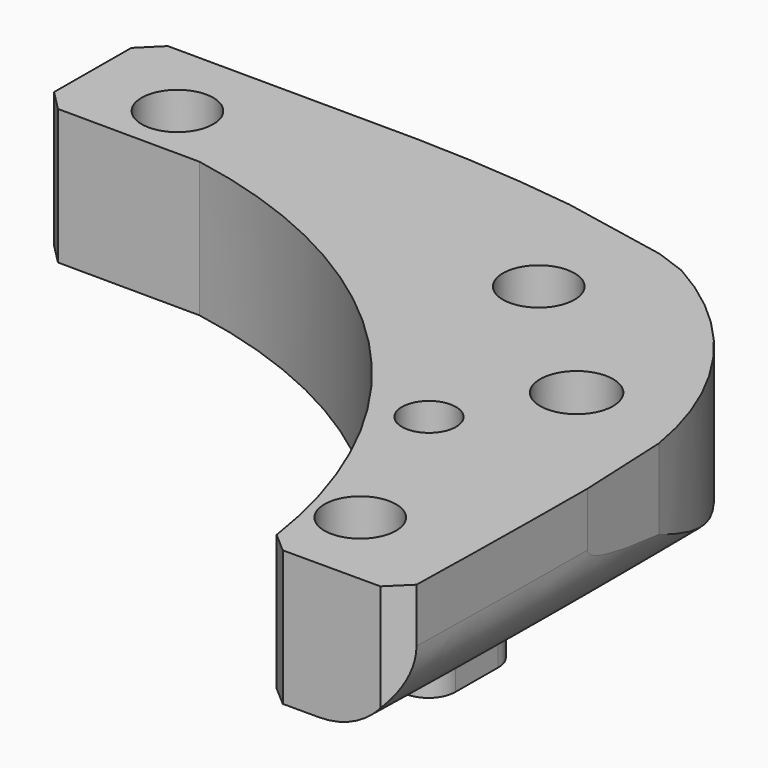
from build123d import *

# Parameters (mm, degrees)
F1_DEPTH    = 10
F2_R        = 2.65
F2_R_2      = 2.7
F3_DEPTH    = 10.001
F4_T2_ANGLE = 6.3743045961
F6_DEPTH    = 6
F7_R        = 2
F8_T1_DEPTH = 17.7150489639
F8_T3_DEPTH = 16.827176909
F8_T5_DEPTH = 14.1871505468
F9_T1_DEPTH = 16.8101610382
F10_R       = 2
F11_DEPTH   = 16


# Not quite as in the source:
# - a fillet or chamfer that OpenCascade refuses, or shapes differently, is made with other operations: its cross-section is extruded or revolved along the edge and cut away or added
# - a feature names something its author has since deleted; it is built from what else it names


with BuildPart() as f1:
    # F0 (on Top) → F1 (new body)
    with BuildSketch(Plane.XY):
        with BuildLine():
            Line((-34.7499609253, -11.2477834763), (-54.7499609253, -11.1477834763))
            Line((-54.7499609253, -11.1477834763), (-54.8004609253, -21.2477834763))
            Line((-54.8004609253, -21.2477834763), (-42.8006109225, -21.3077827264))
            ThreePointArc((-42.8006109225, -21.3077827264), (-20.5885311059, -33.3218659489), (-10, -56.2477834763))
            Line((-10, -56.2477834763), (0, -56.2477834763))
            ThreePointArc((0, -56.2477834763), (0.1673692192, -47.7484327866), (0.2444140549, -39.2477834763))
            Line((0.2444140549, -39.2477834763), (-0.07466726, -32.2477834763))
            ThreePointArc((-0.07466726, -32.2477834763), (-4.6744272783, -21.4152799032), (-13.7499609253, -13.9229094565))
            Line((-13.7499609253, -13.9229094565), (-22.7499609253, -12.1477834763))
            ThreePointArc((-22.7499609253, -12.1477834763), (-28.7364107349, -11.5171142711), (-34.7499609253, -11.2477834763))
        make_face()
    extrude(amount=F1_DEPTH)

    # F2 (on face) → F3 (cut, through all)
    with BuildSketch(Plane.XY.offset(10)):
        with Locations((-47.7499609253, -17.1477834763)):
            Circle(F2_R)
        with Locations((-17.7499609253, -21.2477834763)):
            Circle(F2_R)
        with Locations((-7.7499609253, -50.2477834763)):
            Circle(F2_R)
        with Locations((-7.7499609253, -30.2477834763)):
            Circle(F2_R_2)
    extrude(amount=-F3_DEPTH, mode=Mode.SUBTRACT)

    # F4: fillet of radius 6 on 1 edges, made by hand

    # F4_s1 → F4_t2 (revolve, cut)
    with BuildSketch(Plane(origin=(-6.441827323, -91.8723118046, 0), x_dir=(0, 0, 1), z_dir=(-0.0699454492, -0.9975508178, 0))):
        with BuildLine():
            ThreePointArc((0, 1.2558600799), (1.7573593129, -2.9867806073), (6, -4.7441399201))
            Line((6, -4.7441399201), (6, -4.8641399201))
            Line((6, -4.8641399201), (-0.12, -4.8641399201))
            Line((-0.12, -4.8641399201), (-0.12, 1.2558600799))
            Line((-0.12, 1.2558600799), (0, 1.2558600799))
        make_face()
    revolve(axis=Axis((-799.7499609255, -36.2477834763, 0), (0, 0, 1)), revolution_arc=F4_T2_ANGLE, mode=Mode.SUBTRACT)

    # F5 (on face) → F6 (join)
    with BuildSketch(Plane.XY):
        Polygon((-20, -32.2477834763), (-14.04, -41.3386925673), (-9.04, -42.2477834763), (-9, -34.2477834763), align=None)
    extrude(amount=-F6_DEPTH)

    # F7
    f7_edges = [f1.edges().sort_by_distance(p)[0] for p in [
        (-9, -34.247783, -3),
        (-20, -32.247783, -3),
        (-14.04, -41.338693, -3),
        (-9.04, -42.247783, -3),
    ]]
    fillet(f7_edges, radius=F7_R)

    # F8: chamfer of 1.5 on 4 edges, made by hand

    # F8_s2 → F8_t1 (cut)
    with BuildSketch(Plane.XY.offset(-3.8575244819)):
        Polygon((-53.2499796749, -11.1552833826), (-54.7574608315, -12.6477647267), (-54.7499609253, -11.1477834763), align=None)
        Polygon((-54.792961019, -19.747802226), (-53.3004796749, -21.2552833826), (-54.8004609253, -21.2477834763), align=None)
    extrude(amount=F8_T1_DEPTH, mode=Mode.SUBTRACT)

    # F8_s4 → F8_t3 (cut)
    with BuildSketch(Plane.XY.offset(-3.4135884545)):
        with BuildLine():
            Line((-10.1649915082, -54.9628953089), (-8.6804960049, -56.2477834763))
            Line((-8.6804960049, -56.2477834763), (-10, -56.2477834763))
            ThreePointArc((-10, -56.2477834763), (-10.0801500361, -55.5824778984), (-10.1649915082, -54.9628953089))
        make_face()
    extrude(amount=F8_T3_DEPTH, mode=Mode.SUBTRACT)

    # F8_s6 → F8_t5 (cut)
    with BuildSketch(Plane.XY.offset(-0.4141318258)):
        with BuildLine():
            Line((-1.4642977695, -56.2477834763), (0.0352995939, -54.7825361376))
            ThreePointArc((0.0352995939, -54.7825361376), (0.0185023043, -55.4936979353), (0, -56.2477834763))
            Line((0, -56.2477834763), (-1.4642977695, -56.2477834763))
        make_face()
    extrude(amount=F8_T5_DEPTH, mode=Mode.SUBTRACT)

    # F9: chamfer of 1 on 1 edges, made by hand

    # F9_s2 → F9_t1 (cut)
    with BuildSketch(Plane.XY.offset(-3.4050805191)):
        with BuildLine():
            Line((-12.5377780347, -14.5439926831), (-14.8624749797, -13.6972040173))
            Line((-14.8624749797, -13.6972040173), (-14.8586048158, -13.6775820441))
            ThreePointArc((-14.8586048158, -13.6775820441), (-14.3029436702, -13.7934559205), (-13.7460907615, -13.9032874834))
            Line((-13.7460907615, -13.9032874834), (-13.7412512479, -13.9049055259))
            ThreePointArc((-13.7412512479, -13.9049055259), (-13.1317908034, -14.2101386142), (-12.5281211003, -14.5264785854))
            Line((-12.5281211003, -14.5264785854), (-12.5377780347, -14.5439926831))
        make_face()
    extrude(amount=F9_T1_DEPTH, mode=Mode.SUBTRACT)

    # F10 (on face) → F11 (cut, through all)
    with BuildSketch(Plane(origin=(0, 0, -6), x_dir=(1, 0, 0), z_dir=(0, 0, -1))):
        with Locations((-12.50838816, 37.9476757883)):
            Circle(F10_R)
    extrude(amount=-F11_DEPTH, mode=Mode.SUBTRACT)


solid = f1.part
